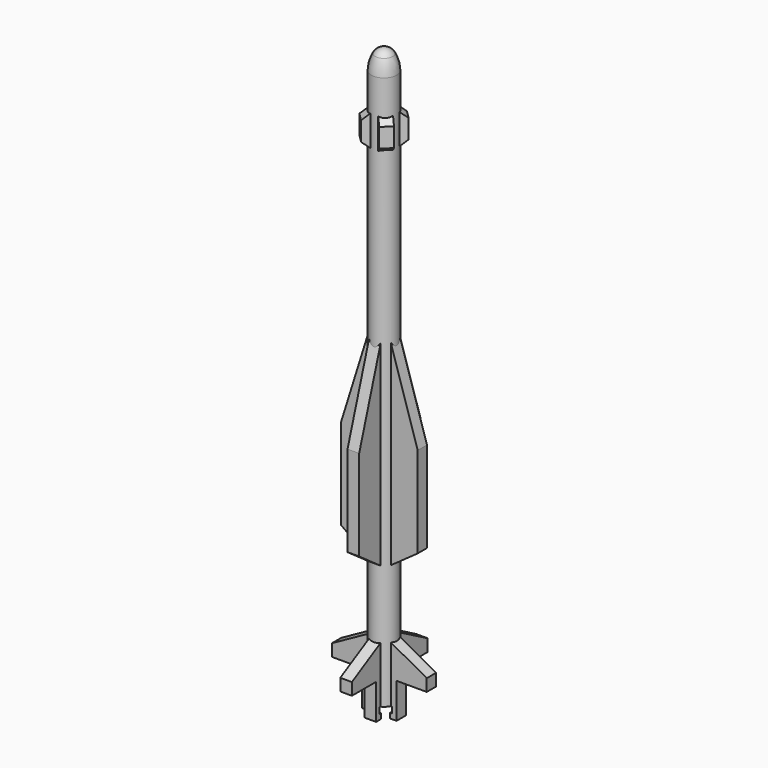
from build123d import *

# Parameters (mm, degrees)
F3_DEPTH = 0.2
F6_DEPTH = 0.2
F7_COUNT = 4


# Not quite as in the source:
# - a feature names something its author has since deleted; it is built from what else it names


with BuildPart() as f1:
    # F0 (on Front) → F1 (revolve)
    with BuildSketch(Plane.XZ):
        with BuildLine():
            Line((0, 19.7569444444), (0, 0))
            Line((0, 0), (0.4409722222, 0))
            Line((0.4409722222, 0), (0.4409722222, 19.0625))
            ThreePointArc((0.4409722222, 19.0625), (0.4053949582, 19.3321442616), (0.3010981711, 19.5833333333))
            ThreePointArc((0.3010981711, 19.5833333333), (0.1737821384, 19.7104325641), (0, 19.7569444444))
        make_face()
    revolve(axis=Axis((0, 0, 9.8784722222), (0, 0, 1)))

    # F2 (on Front) → F3 (join, symmetric)
    with BuildSketch(Plane.XZ):
        Polygon((0, 12.279863856), (0, 3.9918203777), (1.3194444444, 4.9305555556), (1.3194444444, 8.0555555556), align=None)
        Polygon((0, 2.1539925494), (0, 0), (0.4409722222, 0), (0.4409722222, -0.2083333333), (0.3715277778, -0.2083333333), (0.3715277778, -0.3819444444), (0.5902777778, -0.3819444444), (0.5902777778, 0.8333333333), (1.6319444444, 0.8333333333), (1.6319444444, 1.25), align=None)
    extrude(amount=F3_DEPTH, both=True)

    # F5 (on face) → F6 (join, symmetric)
    with BuildSketch(Plane(origin=(0, 0, 0), x_dir=(0.7071067812, -0.7071067812, 0), z_dir=(-0.7071067812, -0.7071067812, 0))):
        Polygon((0, 16.5328663793), (0.6423611111, 17.03125), (0.6423611111, 17.6909722222), (0, 18.1893558429), align=None)
    extrude(amount=F6_DEPTH, both=True)

    # F7: F1 ×4 about axis
    f7_axis = Axis((0, 0, 0), (0, 0, 1))


with BuildPart() as f1_1:
    add(f1.part)
    for i in range(1, F7_COUNT):
        add(f1.part.rotate(f7_axis, i * 360 / F7_COUNT))


solid = f1_1.part
